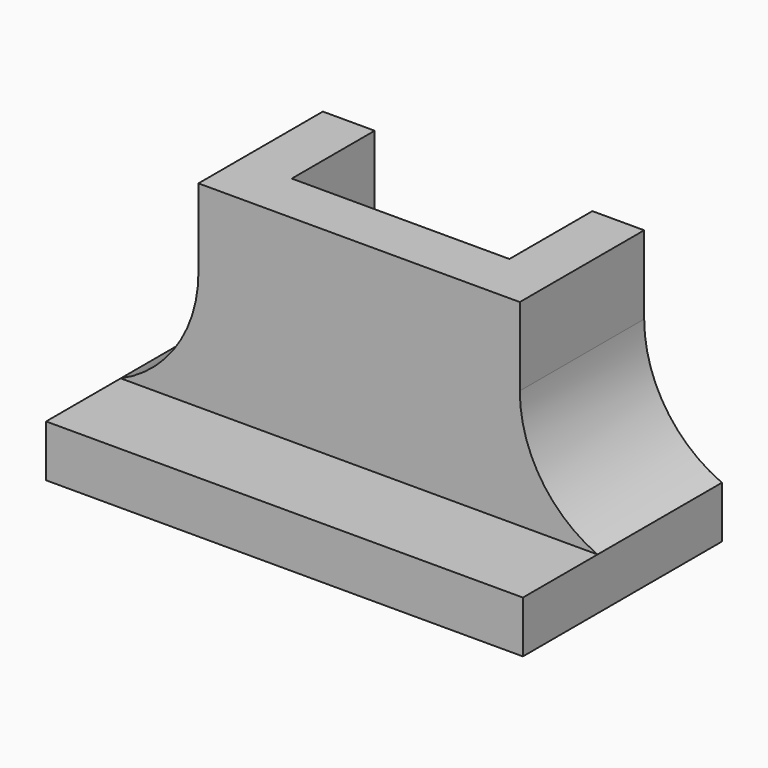
from build123d import *

# Parameters (mm, degrees)
F0_W        = 15
F0_H        = 30
F1_DEPTH    = 48
F2_DEPTH    = 10
F3_W        = 15
F3_H        = 30
F4_DEPTH    = 38
F5_T1_DEPTH = 30


# Not quite as in the source:
# - a fillet or chamfer that OpenCascade refuses, or shapes differently, is made with other operations: its cross-section is extruded or revolved along the edge and cut away or added


with BuildPart() as f1:
    # F0 (on Top) → F1 (new body)
    with BuildSketch(Plane.XY):
        Polygon((21, 0), (0, 0), (-21, 0), (-21, 20), (-31, 20), (-31, -10), (31, -10), (31, 20), (21, 20), align=None)
        with Locations((38.5, 5)):
            Rectangle(F0_W, F0_H)
        with Locations((-38.5, 5)):
            Rectangle(F0_W, F0_H)
    extrude(amount=F1_DEPTH)

    # F0 (on Top) → F2 (join)
    with BuildSketch(Plane.XY):
        Polygon((46, -10), (31, -10), (-31, -10), (-46, -10), (-46, -28), (46, -28), align=None)
    extrude(amount=F2_DEPTH)

    # F3 (on face) → F4 (cut)
    with BuildSketch(Plane.XY.offset(48)):
        with Locations((-38.5, 5)):
            Rectangle(F3_W, F3_H)
        with Locations((38.5, 5)):
            Rectangle(F3_W, F3_H)
    extrude(amount=-F4_DEPTH, mode=Mode.SUBTRACT)

    # F5: fillet of radius 25 on 2 edges, made by hand

    # F5_s2 → F5_t1 (join)
    with BuildSketch(Plane.XZ.offset(-20)):
        with BuildLine():
            ThreePointArc((46, 10), (35.0834993366, 19.2198145372), (31, 32.9128784748))
            Line((31, 32.9128784748), (31, 10))
            Line((31, 10), (46, 10))
        make_face()
        with BuildLine():
            ThreePointArc((-46, 10), (-35.0834993366, 19.2198145372), (-31, 32.9128784748))
            Line((-31, 32.9128784748), (-31, 10))
            Line((-31, 10), (-46, 10))
        make_face()
    extrude(amount=F5_T1_DEPTH)


solid = f1.part
